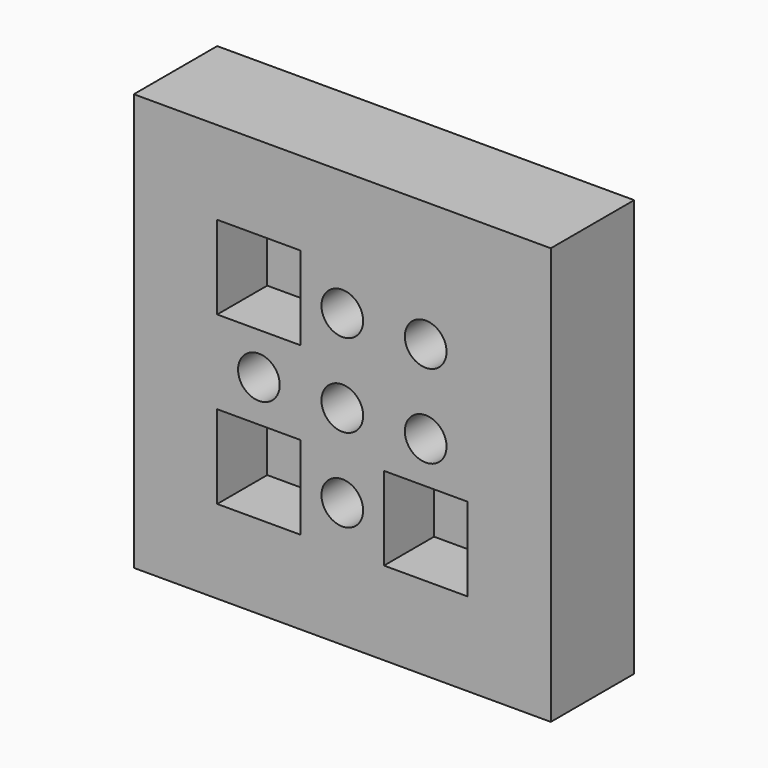
from build123d import *

# Parameters (mm, degrees)
F0_W     = 31.75
F0_H     = 31.75
F0_W_2   = 6.35
F0_H_2   = 6.35
F0_R     = 1.5875
F1_DEPTH = 7.9375
F2_DEPTH = 3.175


# Not quite as in the source:
# - a length typed as a fraction of an inch, garbled in the dataset ("3 / 203.2 mm" for 3/8 in), is restored


with BuildPart() as f1:
    # F0 (on Front) → F1 (new body)
    with BuildSketch(Plane.XZ):
        Rectangle(F0_W, F0_H)
        with Locations((-6.35, -6.35)):
            Rectangle(F0_W_2, F0_H_2, mode=Mode.SUBTRACT)
        with Locations((0, -6.35)):
            Circle(F0_R, mode=Mode.SUBTRACT)
        with Locations((6.35, -6.35)):
            Rectangle(F0_W_2, F0_H_2, mode=Mode.SUBTRACT)
        with Locations((-6.35, 0)):
            Circle(F0_R, mode=Mode.SUBTRACT)
        with Locations((-6.35, 6.35)):
            Rectangle(F0_W_2, F0_H_2, mode=Mode.SUBTRACT)
        Circle(F0_R, mode=Mode.SUBTRACT)
        with Locations((6.35, 0)):
            Circle(F0_R, mode=Mode.SUBTRACT)
        with Locations((0, 6.35)):
            Circle(F0_R, mode=Mode.SUBTRACT)
        with Locations((6.35, 6.35)):
            Circle(F0_R, mode=Mode.SUBTRACT)
    extrude(amount=F1_DEPTH)

    # F0 (on Front) → F2 (join)
    with BuildSketch(Plane.XZ):
        Rectangle(F0_W, F0_H)
        with Locations((-6.35, -6.35)):
            Rectangle(F0_W_2, F0_H_2, mode=Mode.SUBTRACT)
        with Locations((0, -6.35)):
            Circle(F0_R, mode=Mode.SUBTRACT)
        with Locations((6.35, -6.35)):
            Rectangle(F0_W_2, F0_H_2, mode=Mode.SUBTRACT)
        with Locations((-6.35, 0)):
            Circle(F0_R, mode=Mode.SUBTRACT)
        with Locations((-6.35, 6.35)):
            Rectangle(F0_W_2, F0_H_2, mode=Mode.SUBTRACT)
        Circle(F0_R, mode=Mode.SUBTRACT)
        with Locations((6.35, 0)):
            Circle(F0_R, mode=Mode.SUBTRACT)
        with Locations((0, 6.35)):
            Circle(F0_R, mode=Mode.SUBTRACT)
        with Locations((6.35, 6.35)):
            Circle(F0_R, mode=Mode.SUBTRACT)
        with Locations((6.35, -6.35)):
            Rectangle(F0_W_2, F0_H_2)
        with Locations((-6.35, -6.35)):
            Rectangle(F0_W_2, F0_H_2)
        with Locations((-6.35, 6.35)):
            Rectangle(F0_W_2, F0_H_2)
        with Locations((-6.35, 0)):
            Circle(F0_R)
        Circle(F0_R)
        with Locations((0, -6.35)):
            Circle(F0_R)
        with Locations((6.35, 0)):
            Circle(F0_R)
        with Locations((6.35, 6.35)):
            Circle(F0_R)
        with Locations((0, 6.35)):
            Circle(F0_R)
    extrude(amount=F2_DEPTH)


solid = f1.part
